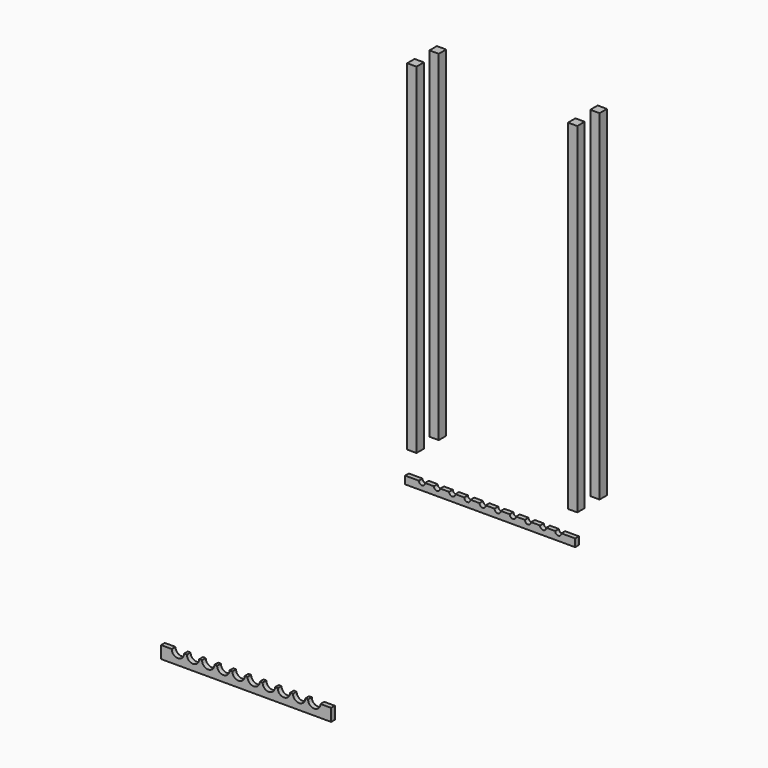
from build123d import *

# Parameters (mm, degrees)
F0_W     = 60
F0_H     = 60
F1_DEPTH = 2200
F3_DEPTH = 30


# Not quite as in the source:
# - a feature names something its author has since deleted; it is built from what else it names


with BuildPart() as f1:
    # F0 (on Top) → F1 (new body)
    with BuildSketch(Plane.XY):
        with Locations((-520, -90)):
            Rectangle(F0_W, F0_H)
    extrude(amount=F1_DEPTH)


with BuildPart() as f1b:
    # F0 (on Top) → F1, piece 2 (new body)
    with BuildSketch(Plane.XY):
        with Locations((520, -90)):
            Rectangle(F0_W, F0_H)
    extrude(amount=F1_DEPTH)


with BuildPart() as f1c:
    # F0 (on Top) → F1, piece 3 (new body)
    with BuildSketch(Plane.XY):
        with Locations((520, 90)):
            Rectangle(F0_W, F0_H)
    extrude(amount=F1_DEPTH)


with BuildPart() as f1d:
    # F0 (on Top) → F1, piece 4 (new body)
    with BuildSketch(Plane.XY):
        with Locations((-520, 90)):
            Rectangle(F0_W, F0_H)
    extrude(amount=F1_DEPTH)


with BuildPart() as f3:
    # F2 (on Front) → F3 (new body)
    with BuildSketch(Plane.XZ):
        with BuildLine():
            Line((464.1985823002, -212.5107118107), (375.1985823002, -212.5107118107))
            ThreePointArc((375.1985823002, -212.5107118107), (355.1985823002, -232.5107118107), (335.1985823002, -212.5107118107))
            Line((335.1985823002, -212.5107118107), (277.1985823002, -212.5107118107))
            ThreePointArc((277.1985823002, -212.5107118107), (257.1985823002, -232.5107118107), (237.1985823002, -212.5107118107))
            Line((237.1985823002, -212.5107118107), (179.1985823002, -212.5107118107))
            ThreePointArc((179.1985823002, -212.5107118107), (159.1985823002, -232.5107118107), (139.1985823002, -212.5107118107))
            Line((139.1985823002, -212.5107118107), (81.1985823002, -212.5107118107))
            ThreePointArc((81.1985823002, -212.5107118107), (61.1985823002, -232.5107118107), (41.1985823002, -212.5107118107))
            Line((41.1985823002, -212.5107118107), (-16.8014176998, -212.5107118107))
            ThreePointArc((-16.8014176998, -212.5107118107), (-36.8014176998, -232.5107118107), (-56.8014176998, -212.5107118107))
            Line((-56.8014176998, -212.5107118107), (-114.8014176998, -212.5107118107))
            ThreePointArc((-114.8014176998, -212.5107118107), (-134.8014176998, -232.5107118107), (-154.8014176998, -212.5107118107))
            Line((-154.8014176998, -212.5107118107), (-212.8014176998, -212.5107118107))
            ThreePointArc((-212.8014176998, -212.5107118107), (-232.8014176998, -232.5107118107), (-252.8014176998, -212.5107118107))
            Line((-252.8014176998, -212.5107118107), (-310.8014176998, -212.5107118107))
            ThreePointArc((-310.8014176998, -212.5107118107), (-330.8014176998, -232.5107118107), (-350.8014176998, -212.5107118107))
            Line((-350.8014176998, -212.5107118107), (-408.8014176998, -212.5107118107))
            ThreePointArc((-408.8014176998, -212.5107118107), (-428.8014176998, -232.5107118107), (-448.8014176998, -212.5107118107))
            Line((-448.8014176998, -212.5107118107), (-506.8014176998, -212.5107118107))
            ThreePointArc((-506.8014176998, -212.5107118107), (-526.8014176998, -232.5107118107), (-546.8014176998, -212.5107118107))
            Line((-546.8014176998, -212.5107118107), (-635.8014176998, -212.5107118107))
            Line((-635.8014176998, -212.5107118107), (-635.8014176998, -262.5107118107))
            Line((-635.8014176998, -262.5107118107), (464.1985823002, -262.5107118107))
            Line((464.1985823002, -262.5107118107), (464.1985823002, -212.5107118107))
        make_face()
    extrude(amount=F3_DEPTH)


with BuildPart() as f3b:
    # F2 (on Front) → F3, piece 2 (new body)
    with BuildSketch(Plane.XZ):
        with BuildLine():
            Line((-1114.0999228668, -1690.6479753494), (-1183.0999228668, -1690.6479753494))
            ThreePointArc((-1183.0999228668, -1690.6479753494), (-1223.0999228668, -1730.6479753494), (-1263.0999228668, -1690.6479753494))
            Line((-1263.0999228668, -1690.6479753494), (-1281.0999228668, -1690.6479753494))
            ThreePointArc((-1281.0999228668, -1690.6479753494), (-1321.0999228668, -1730.6479753494), (-1361.0999228668, -1690.6479753494))
            Line((-1361.0999228668, -1690.6479753494), (-1379.0999228668, -1690.6479753494))
            ThreePointArc((-1379.0999228668, -1690.6479753494), (-1419.0999228668, -1730.6479753494), (-1459.0999228668, -1690.6479753494))
            Line((-1459.0999228668, -1690.6479753494), (-1477.0999228668, -1690.6479753494))
            ThreePointArc((-1477.0999228668, -1690.6479753494), (-1517.0999228668, -1730.6479753494), (-1557.0999228668, -1690.6479753494))
            Line((-1557.0999228668, -1690.6479753494), (-1575.0999228668, -1690.6479753494))
            ThreePointArc((-1575.0999228668, -1690.6479753494), (-1615.0999228668, -1730.6479753494), (-1655.0999228668, -1690.6479753494))
            Line((-1655.0999228668, -1690.6479753494), (-1673.0999228668, -1690.6479753494))
            ThreePointArc((-1673.0999228668, -1690.6479753494), (-1713.0999228668, -1730.6479753494), (-1753.0999228668, -1690.6479753494))
            Line((-1753.0999228668, -1690.6479753494), (-1771.0999228668, -1690.6479753494))
            ThreePointArc((-1771.0999228668, -1690.6479753494), (-1811.0999228668, -1730.6479753494), (-1851.0999228668, -1690.6479753494))
            Line((-1851.0999228668, -1690.6479753494), (-1869.0999228668, -1690.6479753494))
            ThreePointArc((-1869.0999228668, -1690.6479753494), (-1909.0999228668, -1730.6479753494), (-1949.0999228668, -1690.6479753494))
            Line((-1949.0999228668, -1690.6479753494), (-1967.0999228668, -1690.6479753494))
            ThreePointArc((-1967.0999228668, -1690.6479753494), (-2007.0999228668, -1730.6479753494), (-2047.0999228668, -1690.6479753494))
            Line((-2047.0999228668, -1690.6479753494), (-2065.0999228668, -1690.6479753494))
            ThreePointArc((-2065.0999228668, -1690.6479753494), (-2105.0999228668, -1730.6479753494), (-2145.0999228668, -1690.6479753494))
            Line((-2145.0999228668, -1690.6479753494), (-2214.0999228668, -1690.6479753494))
            Line((-2214.0999228668, -1690.6479753494), (-2214.0999228668, -1770.6479753494))
            Line((-2214.0999228668, -1770.6479753494), (-1114.0999228668, -1770.6479753494))
            Line((-1114.0999228668, -1770.6479753494), (-1114.0999228668, -1690.6479753494))
        make_face()
    extrude(amount=F3_DEPTH)


solid = Compound([f1.part, f1b.part, f1c.part, f1d.part, f3.part, f3b.part])
